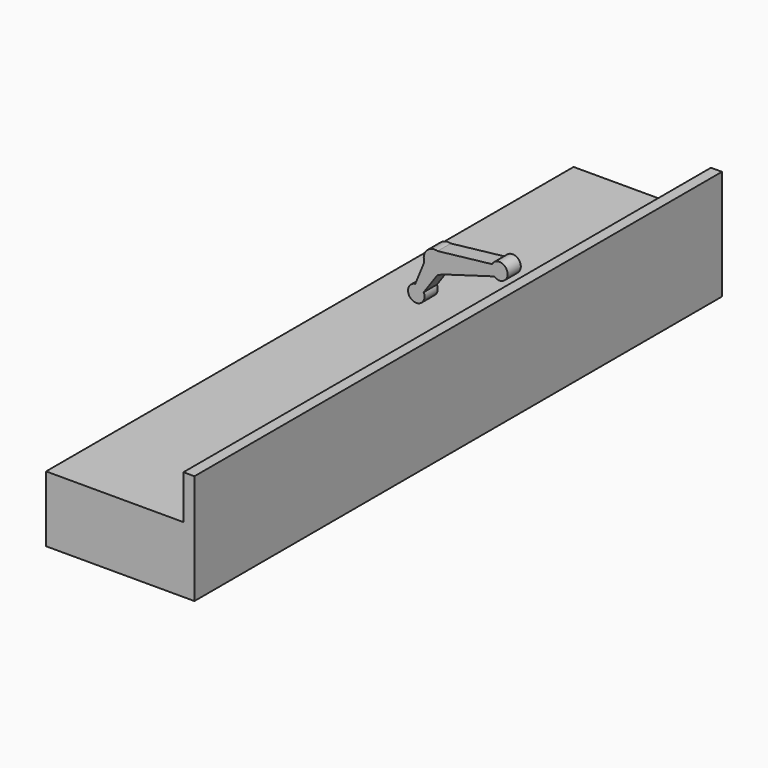
from build123d import *

# Parameters (mm, degrees)
F1_DEPTH = 1524
F3_DEPTH = 38.1


# Not quite as in the source:
# - the program builds the solid bodies; features that only make, move or delete a surface that nothing else refers to are left out


with BuildPart() as f1:
    # F0 (on Front) → F1 (new body, symmetric)
    with BuildSketch(Plane.XZ):
        Polygon((0, 0), (-635, 0), (-635, -304.8), (50.8, -304.8), (50.8, 203.2), (0, 203.2), align=None)
    extrude(amount=F1_DEPTH, both=True)


with BuildPart() as f3:
    # F2 (on Front) → F3 (new body, symmetric)
    with BuildSketch(Plane.XZ):
        with BuildLine():
            ThreePointArc((-75.3569098829, 429.5622010227), (-51.5175746271, 401.0427737637), (-14.6388120751, 396.3921276521))
            ThreePointArc((-14.6388120751, 396.3921276521), (-4.7830646148, 400.019479985), (4.1161927035, 405.5959181074))
            ThreePointArc((4.1161927035, 405.5959181074), (18.4967583285, 423.3568590758), (23.6370308853, 445.6240836405))
            ThreePointArc((23.6370308853, 445.6240836405), (13.220292501, 476.443431156), (-13.7579368817, 494.6235235438))
            ThreePointArc((-13.7579368817, 494.6235235438), (-64.0521404433, 480.5501346438), (-75.3569098829, 429.5622010227))
        make_face()
        with BuildLine():
            ThreePointArc((23.6370308853, 445.6240836405), (18.4967583285, 423.3568590758), (4.1161927035, 405.5959181074))
            Line((4.1161927035, 405.5959181074), (247.2621074291, 476.3695837783))
            ThreePointArc((247.2621074291, 476.3695837783), (234.3190735269, 498.1220014658), (237.8630415532, 523.1845251311))
            Line((237.8630415532, 523.1845251311), (-13.7579368817, 494.6235235438))
            ThreePointArc((-13.7579368817, 494.6235235438), (13.220292501, 476.443431156), (23.6370308853, 445.6240836405))
        make_face()
        with BuildLine():
            ThreePointArc((237.8630415532, 523.1845251311), (234.3190735269, 498.1220014658), (247.2621074291, 476.3695837783))
            ThreePointArc((247.2621074291, 476.3695837783), (287.8218736761, 471.1130832643), (309.7736510471, 505.6217040122))
            ThreePointArc((309.7736510471, 505.6217040122), (280.713169239, 542.6338251465), (237.8630415532, 523.1845251311))
        make_face()
        with BuildLine():
            ThreePointArc((-117.0813960528, 327.4013066613), (-137.6370487848, 261.0429106479), (-74.3040884081, 289.5894990716))
            ThreePointArc((-74.3040884081, 289.5894990716), (-75.2548147797, 298.0477180849), (-78.059546092, 306.0838136404))
            ThreePointArc((-78.059546092, 306.0838136404), (-94.1381342738, 323.0254814792), (-117.0813960528, 327.4013066613))
        make_face()
        with BuildLine():
            ThreePointArc((-117.0813960528, 327.4013066613), (-94.1381342738, 323.0254814792), (-78.059546092, 306.0838136404))
            Line((-78.059546092, 306.0838136404), (-14.6388120751, 396.3921276521))
            ThreePointArc((-14.6388120751, 396.3921276521), (-51.5175746271, 401.0427737637), (-75.3569098829, 429.5622010227))
            Line((-75.3569098829, 429.5622010227), (-117.0813960528, 327.4013066613))
        make_face()
    extrude(amount=F3_DEPTH, both=True)


solid = Compound([f1.part, f3.part])
